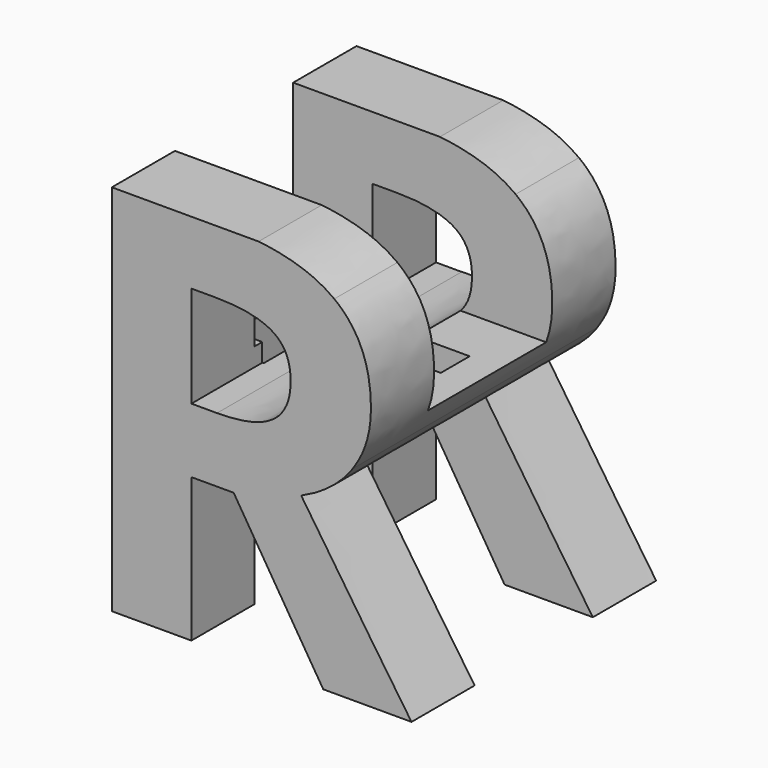
from build123d import *

# Parameters (mm, degrees)
F0_W         = 31.75
F0_H         = 31.75
F1_DEPTH     = 31.75
F3_DEPTH     = 31.751
F4_W         = 12.3424336089
F4_H         = 13.4545489644
F5_DEPTH     = 25.0325832888
F6_TEXT_SIZE = 19.9109252102
F7_DEPTH     = 31.1743440242


# Not quite as in the source:
# - Text() gives the source's letters only with a copy of the font that has no kerning and outlines rounded to 1/6400 em; it was checked with that copy


with BuildPart() as f1:
    # F0 (on Front) → F1 (new body)
    with BuildSketch(Plane.XZ):
        with Locations((15.875, 15.875)):
            Rectangle(F0_W, F0_H)
    extrude(amount=F1_DEPTH)

    # F2 (on face) → F3 (cut, through all)
    with BuildSketch(Plane.XZ.offset(31.75)):
        with BuildLine():
            Line((0, 0), (3.9228874832, 0))
            Line((3.9228874832, 0), (3.9228874832, 31.334055778))
            Line((3.9228874832, 31.334055778), (13.0508428871, 31.334055778))
            add(Edge.make_bspline(
                [(13.0508428871, 31.334055778), (19.4424690603, 31.334055778), (22.5045517709, 29.0092046271)],
                knots=[0, 0, 0, 1, 1, 1], degree=2))
            add(Edge.make_bspline(
                [(22.5045517709, 29.0092046271), (25.5666344815, 26.6843534761), (25.5666344815, 21.9454975902)],
                knots=[0, 0, 0, 1, 1, 1], degree=2))
            add(Edge.make_bspline(
                [(25.5666344815, 21.9454975902), (25.5666344815, 19.1817364875), (24.0475945702, 17.0283345364)],
                knots=[0, 0, 0, 1, 1, 1], degree=2))
            add(Edge.make_bspline(
                [(24.0475945702, 17.0283345364), (22.5285546589, 14.8749325854), (19.7373616841, 13.6542142819)],
                knots=[0, 0, 0, 1, 1, 1], degree=2))
            add(Edge.make_bspline(
                [(19.7373616841, 13.6542142819), (26.814784657, 3.0860855986), (28.954470672, 0)],
                knots=[0, 0, 0, 1, 1, 1], degree=2))
            Line((28.954470672, 0), (31.75, 0))
            Line((31.75, 0), (31.75, 31.75))
            Line((31.75, 31.75), (0, 31.75))
            Line((0, 31.75), (0, 0))
        make_face()
        Polygon((14.1001119907, 12.0220178986), (10.5682584722, 12.0220178986), (10.5682584722, 0), (21.5821550753, 0), align=None)
        with BuildLine():
            Line((10.5682584722, 25.8888291885), (10.5682584722, 17.4260966802))
            Line((10.5682584722, 17.4260966802), (12.7079444873, 17.4260966802))
            add(Edge.make_bspline(
                [(12.7079444873, 17.4260966802), (15.8626097659, 17.4260966802), (17.3610757732, 18.4753657838)],
                knots=[0, 0, 0, 1, 1, 1], degree=2))
            add(Edge.make_bspline(
                [(17.3610757732, 18.4753657838), (18.8595417805, 19.5246348873), (18.8595417805, 21.7740483903)],
                knots=[0, 0, 0, 1, 1, 1], degree=2))
            add(Edge.make_bspline(
                [(18.8595417805, 21.7740483903), (18.8595417805, 24.0028879893), (17.3267859332, 24.9458585889)],
                knots=[0, 0, 0, 1, 1, 1], degree=2))
            add(Edge.make_bspline(
                [(17.3267859332, 24.9458585889), (15.7940300859, 25.8888291885), (12.5845010633, 25.8888291885)],
                knots=[0, 0, 0, 1, 1, 1], degree=2))
            Line((12.5845010633, 25.8888291885), (10.5682584722, 25.8888291885))
        make_face()
    extrude(amount=-F3_DEPTH, mode=Mode.SUBTRACT)

    # F4 (on face) → F5 (cut, through all)
    with BuildSketch(Plane(origin=(3.9228874832, 0, 0), x_dir=(0, -1, 0), z_dir=(-1, 0, 0))):
        Polygon((28.6028820729, 31.1733439242), (28.6028820729, 0), (31.75, 0), (31.75, 31.334055778), (0, 31.334055778), (0, 0), (3.0583428626, 0), (3.0583428626, 31.1733439242), (9.6696298537, 31.1733439242), (9.6696298537, 18.9537206), (22.0120634626, 18.9537206), (22.0120634626, 31.1733439242), align=None)
        with Locations((15.8408466581, 6.7272744822)):
            Rectangle(F4_W, F4_H)
    extrude(amount=-F5_DEPTH, mode=Mode.SUBTRACT)

    # F6 (on face) → F7 (cut, through all)
    with BuildSketch(Plane.XY.offset(31.1733439242)):
        with Locations(Location((22.3915317171, -21.6037945718), (0, 0, 90))):
            Text('T', F6_TEXT_SIZE, font='Open Sans', font_style=FontStyle.BOLD, text_align=(TextAlign.LEFT, TextAlign.BOTTOM))
    extrude(amount=-F7_DEPTH, mode=Mode.SUBTRACT)


solid = f1.part
